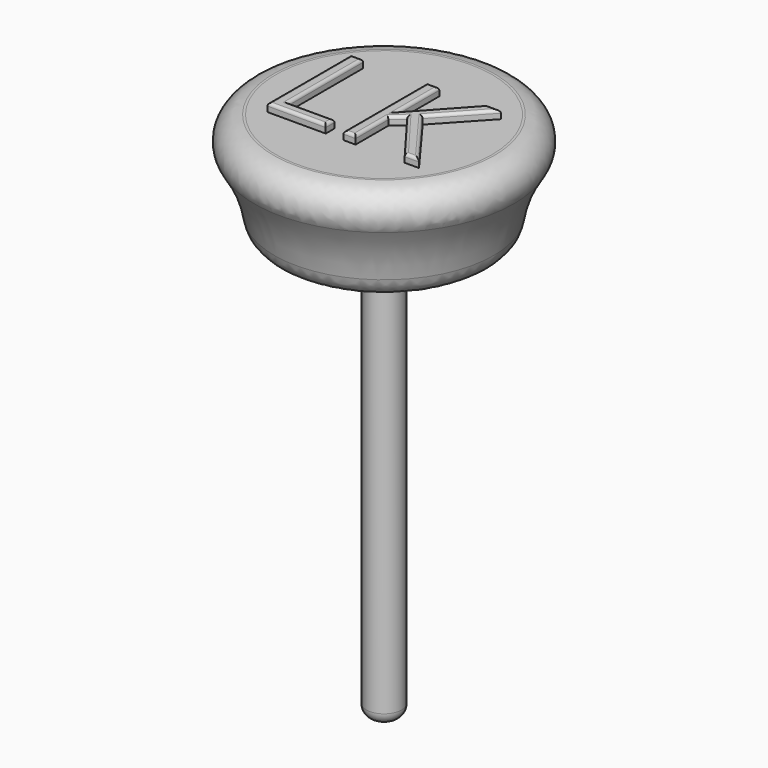
from build123d import *

# Parameters (mm, degrees)
F2_TEXT_SIZE = 25.0489236791
F3_DEPTH     = 19.9
F4_R         = 4
F5_R         = 2
F6_R         = 0.5


# Not quite as in the source:
# - Text() gives the source's letters only with a copy of the font that has no kerning and outlines rounded to 1/6400 em; it was checked with that copy


with BuildPart() as f1:
    # F0 (on Front) → F1 (revolve)
    with BuildSketch(Plane.XZ):
        with BuildLine():
            ThreePointArc((7.5064527399, 0), (7.836931039, 0.0112778063), (8.1674093381, 0))
            Line((8.1674093381, 0), (18.5, 0))
            Line((18.5, 0), (18.5, 18.4999981535))
            Line((18.5, 18.4999981535), (0, 18.4999981535))
            Line((0, 18.4999981535), (0, 0))
            Line((0, 0), (0, -72.144754231))
            Line((0, -72.144754231), (3.0140471645, -72.144754231))
            Line((3.0140471645, -72.144754231), (3.0140471645, -4.3464386836))
            Line((3.0140471645, -4.3464386836), (3.0140471645, 0))
            Line((3.0140471645, 0), (7.5064527399, 0))
        make_face()
        with BuildLine():
            Line((7.5064527399, 0), (8.1674093381, 0))
            ThreePointArc((8.1674093381, 0), (7.836931039, 0.0112778063), (7.5064527399, 0))
        make_face()
        with BuildLine():
            Line((18.5, 18.4999981535), (18.5, 0))
            ThreePointArc((18.5, 0), (21.1087103228, 10.4506255849), (28.3227711916, 18.4492673725))
            Line((28.3227711916, 18.4492673725), (18.5, 18.4999981535))
        make_face()
        with BuildLine():
            ThreePointArc((3.0140471645, -4.3464386836), (4.4661495672, -1.3524506029), (7.5064527399, 0))
            Line((7.5064527399, 0), (3.0140471645, 0))
            Line((3.0140471645, 0), (3.0140471645, -4.3464386836))
        make_face()
    revolve(axis=Axis((0, 0, -23.5352199525), (0, 0, -1)))

    # F2 (on Top) → F3 (join)
    with BuildSketch(Plane.XY):
        with Locations((-15.0748560753, -9.1497124876)):
            Text('LK', F2_TEXT_SIZE, font='Open Sans', text_align=(TextAlign.LEFT, TextAlign.BOTTOM))
    extrude(amount=F3_DEPTH)

    # F4
    f4_edges = [f1.edges().sort_by_distance(p)[0] for p in [
        (-18.5, 0, 0),
        (-28.322771, 0, 18.449267),
    ]]
    fillet(f4_edges, radius=F4_R)

    # F5
    f5_edges = [f1.edges().sort_by_distance(p)[0] for p in [
        (-3.014047, 0, -72.144754),
    ]]
    fillet(f5_edges, radius=F5_R)

    # F6
    f6_edges = [f1.edges().sort_by_distance(p)[0] for p in [
        (-7.632586, -9.149712, 19.9),
        (-12.61693, -0.208421, 19.9),
        (-10.538653, 0.732871, 19.9),
        (-2.648242, -8.208421, 19.9),
        (-6.593447, -7.267129, 19.9),
        (-11.577791, 8.732871, 19.9),
        (1.424165, 8.732871, 19.9),
        (2.463304, 4.298428, 19.9),
        (0.385027, -0.208421, 19.9),
        (2.463304, -5.64482, 19.9),
        (1.424165, -9.149712, 19.9),
        (3.400682, -1.308225, 19.9),
        (6.518099, 4.298428, 19.9),
        (11.801856, 8.732871, 19.9),
        (9.435907, 4.848331, 19.9),
        (9.570936, -4.092961, 19.9),
        (12.077786, -9.149712, 19.9),
        (7.596377, -4.813118, 19.9),
    ]]
    fillet(f6_edges, radius=F6_R)


solid = f1.part
